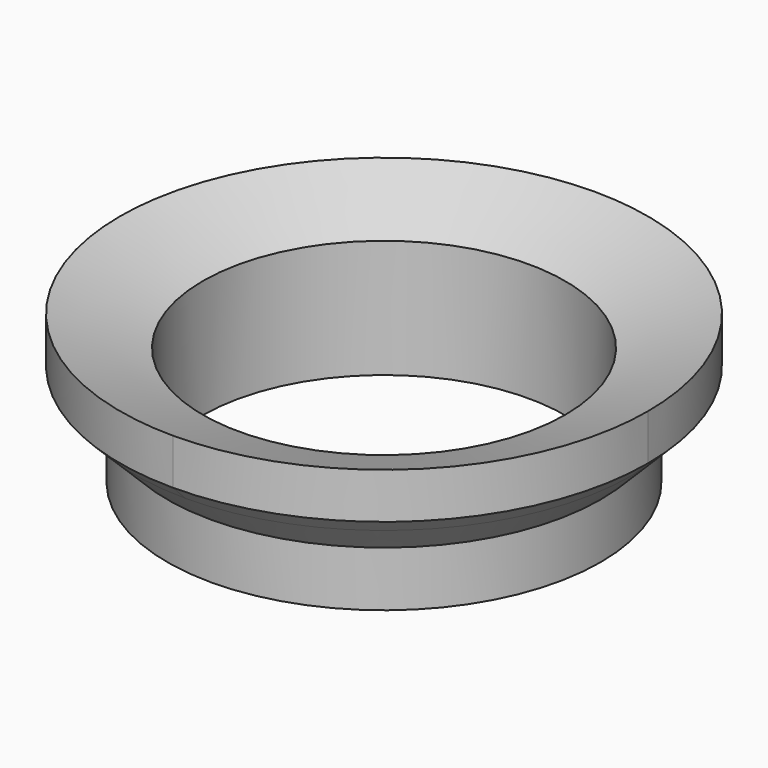
from build123d import *

# Parameters (mm, degrees)
F0_R     = 13.75
F0_R_2   = 11.5
F1_DEPTH = 8.4
F3_R     = 11.5
F4_DEPTH = 4
F6_SIZE  = 2
F7_SIZE  = 0.99999


# Not quite as in the source:
# - a fillet or chamfer that OpenCascade refuses, or shapes differently, is made with other operations: its cross-section is extruded or revolved along the edge and cut away or added
# - a fillet or chamfer is up to 0.001 mm smaller than in the source, because OpenCascade refuses the exact size


with BuildPart() as f1:
    # F0 (on Top) → F1 (new body)
    with BuildSketch(Plane.XY):
        Circle(F0_R)
        Circle(F0_R_2, mode=Mode.SUBTRACT)
    extrude(amount=F1_DEPTH)

    # F3 (on offset) → F4 (join)
    with BuildSketch(Plane.XY.offset(5.5)):
        with BuildLine():
            ThreePointArc((-16.75, 0), (-11.8440385849, -11.8440385849), (0, -16.75))
            ThreePointArc((0, -16.75), (11.8440385849, -11.8440385849), (16.75, 0))
            ThreePointArc((16.75, 0), (11.8440385849, 11.8440385849), (0, 16.75))
            ThreePointArc((0, 16.75), (-11.8440385849, 11.8440385849), (-16.75, 0))
        make_face()
        Circle(F3_R, mode=Mode.SUBTRACT)
    extrude(amount=F4_DEPTH)

    # F5: chamfer of 2 x 5.4949548389 on 1 edges, made by hand

    # F5_s1 → F5_t2 (revolve, cut)
    with BuildSketch(Plane.XZ):
        Polygon((16.9949548389, 9.5), (11.5, 7.5), (11.5, 9.5), align=None)
    revolve(axis=Axis((0, 0, 9.5), (0, 0, 1)), mode=Mode.SUBTRACT)

    # F6
    f6_edges = [f1.edges().sort_by_distance(p)[0] for p in [
        (-13.75, 0, 5.5),
    ]]
    chamfer(f6_edges, length=F6_SIZE)

    # F7 (size 1 in the source; OpenCascade refuses exactly that, so slightly less here)
    f7_edges = [f1.edges().sort_by_distance(p)[0] for p in [
        (0, 16.75, 5.5),
    ]]
    chamfer(f7_edges, length=F7_SIZE)


solid = f1.part
